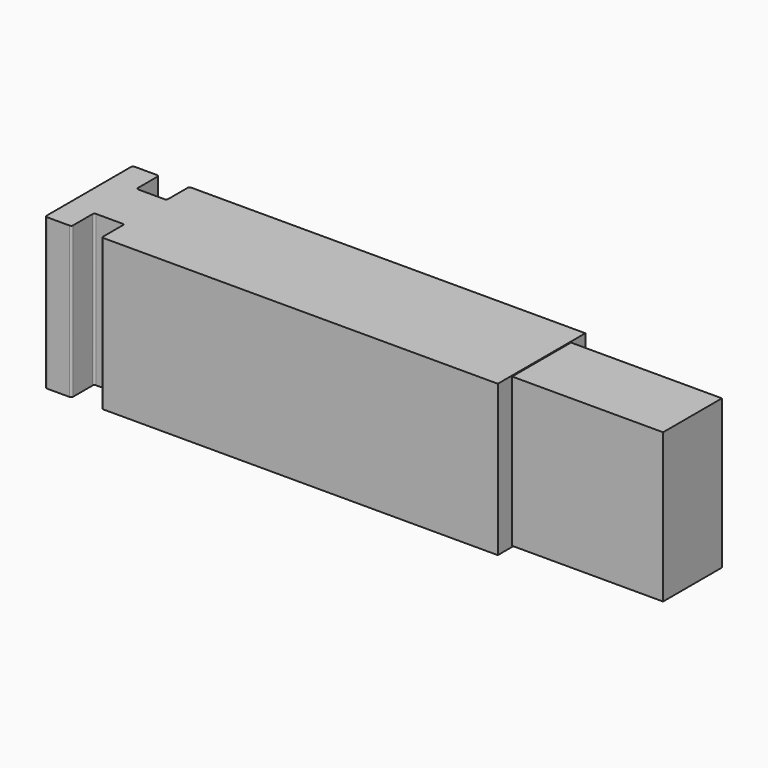
from build123d import *

# Parameters (mm, degrees)
F1_DEPTH = 8
F2_W     = 5.8
F2_H     = 8
F3_DEPTH = 8
F4_R     = 0.1


# Not quite as in the source:
# - a feature names something its author has since deleted; it is built from what else it names


with BuildPart() as f1:
    # F0 (on Top) → F1 (new body)
    with BuildSketch(Plane.XY):
        Polygon((-16.1652290315, 5.6598789893), (-45.1652290315, 5.6598789893), (-45.1652290315, 4.1598789893), (-46.7652290315, 4.1598789893), (-46.7652290315, 5.6598789893), (-48.1652290315, 5.6598789893), (-48.1652290315, -0.1401210107), (-46.7652290315, -0.1401210107), (-46.7652290315, 1.3598789893), (-45.1652290315, 1.3598789893), (-45.1652290315, -0.1401210107), (-16.1652290315, -0.1401210107), align=None)
    extrude(amount=F1_DEPTH)

    # F2 (on face) → F3 (cut)
    with BuildSketch(Plane.YZ.offset(-16.1652290315)):
        with Locations((2.7598789893, 4)):
            Rectangle(F2_W, F2_H)
        Polygon((4.7098789893, 0.05), (2.7598789893, 0.05), (0.8098789893, 0.05), (0.8098789893, 4), (0.8098789893, 7.95), (2.7598789893, 7.95), (4.7098789893, 7.95), (4.7098789893, 4), align=None, mode=Mode.SUBTRACT)
    extrude(amount=-F3_DEPTH, mode=Mode.SUBTRACT)

    # F4
    f4_edges = [f1.edges().sort_by_distance(p)[0] for p in [
        (-46.765229, -0.140121, 4),
        (-46.765229, 1.359879, 4),
        (-46.765229, 4.159879, 4),
        (-46.765229, 5.659879, 4),
        (-48.165229, 5.659879, 4),
        (-48.165229, -0.140121, 4),
        (-45.165229, -0.140121, 4),
        (-45.165229, 5.659879, 4),
        (-45.165229, 4.159879, 4),
        (-45.165229, 1.359879, 4),
    ]]
    fillet(f4_edges, radius=F4_R)


solid = f1.part
